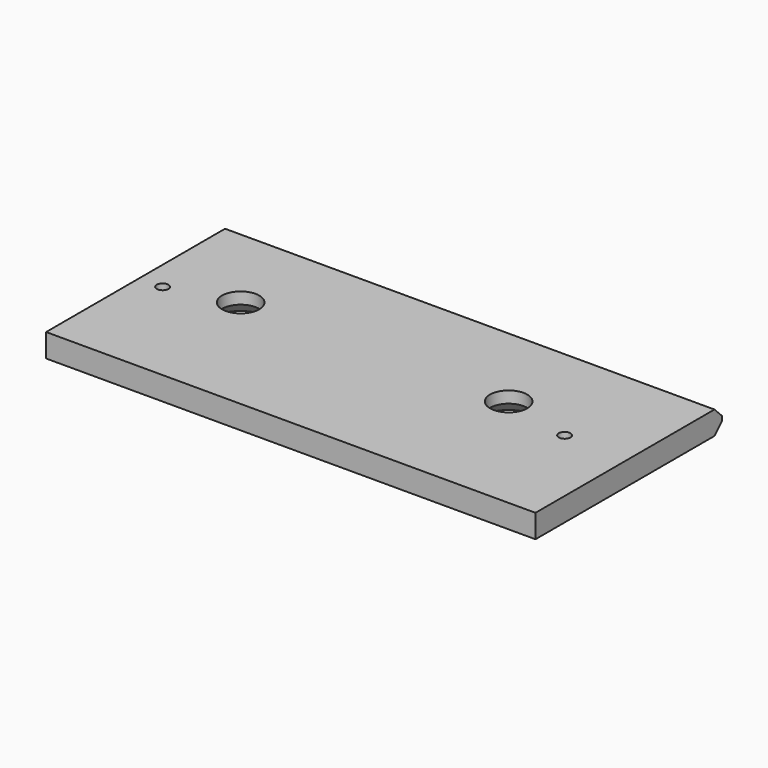
from build123d import *

# Parameters (mm, degrees)
F0_W           = 210
F0_H           = 100
F1_DEPTH       = 10
F2_D           = 5
F2_CSINK_D     = 10
F2_CSINK_ANGLE = 90
F3_D           = 16
F3_CSINK_D     = 26
F3_CSINK_ANGLE = 90
F4_SIZE        = 4


with BuildPart() as f1:
    # F0 (on Top) → F1 (new body)
    with BuildSketch(Plane.XY):
        with Locations((-47.4317967892, 44.5945628711)):
            Rectangle(F0_W, F0_H)
    extrude(amount=F1_DEPTH)

    # F2 (through all)
    with Locations(Plane(origin=(0, 0, 0), x_dir=(1, 0, 0), z_dir=(0, 0, -1))):
        with Locations((30.0682032108, -44.5945628711), (-142.4317967892, -44.5945628711)):
            CounterSinkHole(F2_D / 2, F2_CSINK_D / 2, counter_sink_angle=F2_CSINK_ANGLE)

    # F3 (through all)
    with Locations(Plane(origin=(0, 0, 0), x_dir=(1, 0, 0), z_dir=(0, 0, -1))):
        with Locations((-114.9317967892, -52.0945628711), (0.0682032108, -52.0945628711)):
            CounterSinkHole(F3_D / 2, F3_CSINK_D / 2, counter_sink_angle=F3_CSINK_ANGLE)

    # F4
    f4_edges = [f1.edges().sort_by_distance(p)[0] for p in [
        (-47.431797, 94.594563, 0),
        (-47.431797, 94.594563, 10),
    ]]
    chamfer(f4_edges, length=F4_SIZE)


solid = f1.part
